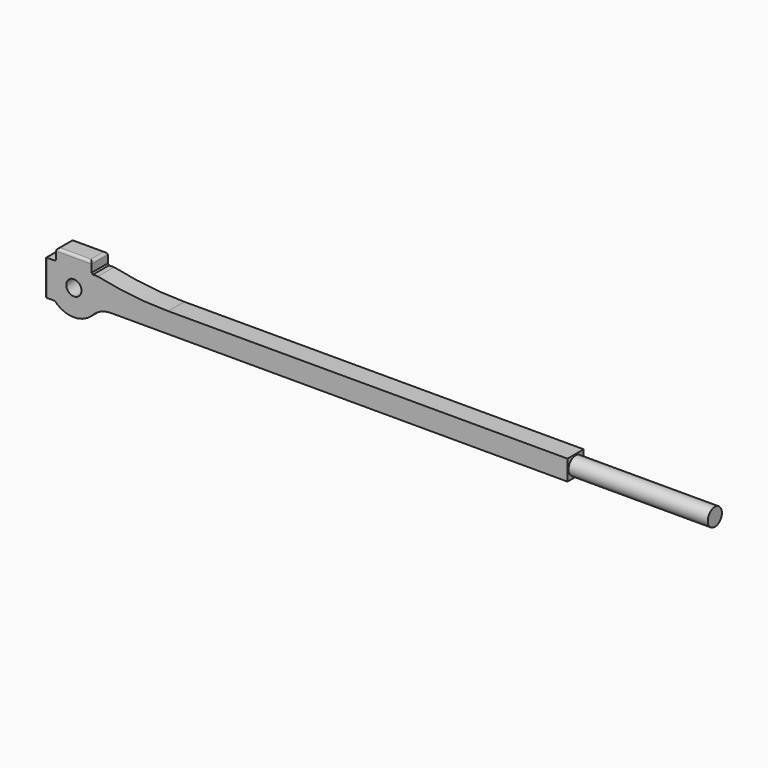
from build123d import *

# Parameters (mm, degrees)
F0_R        = 3
F1_DEPTH    = 8
F2_R        = 10
F3_T1_DEPTH = 8
F4_R        = 1
F5_R        = 3.5
F6_DEPTH    = 55


# Not quite as in the source:
# - a fillet or chamfer that OpenCascade refuses, or shapes differently, is made with other operations: its cross-section is extruded or revolved along the edge and cut away or added


with BuildPart() as f1:
    # F0 (on Front) → F1 (new body)
    with BuildSketch(Plane.XZ):
        with BuildLine():
            Line((-7.5, 7), (-11.5, 7))
            Line((-11.5, 7), (-11.5, -7))
            Line((-11.5, -7), (-7.5, -7))
            ThreePointArc((-7.5, -7), (0, -10.2591422643), (7.5, -7))
            ThreePointArc((7.5, -7), (8.6053519278, -5.5855096632), (9.4472218138, -4))
            Line((9.4472218138, -4), (9.5, -4))
            Line((9.5, -4), (195, -4))
            Line((195, -4), (195, 4))
            Line((195, 4), (9.5, 4))
            Line((9.5, 4), (9.5, 7))
            Line((9.5, 7), (7.5, 7))
            ThreePointArc((7.5, 7), (7.2543090643, 7.2543090643), (7, 7.5))
            Line((7, 7.5), (7, 11.5))
            Line((7, 11.5), (-7, 11.5))
            Line((-7, 11.5), (-7, 7.5))
            ThreePointArc((-7, 7.5), (-7.2543090643, 7.2543090643), (-7.5, 7))
        make_face()
        Circle(F0_R, mode=Mode.SUBTRACT)
    extrude(amount=F1_DEPTH)

    # F2
    f2_edges = [f1.edges().sort_by_distance(p)[0] for p in [
        (9.447222, -4, -4),
    ]]
    fillet(f2_edges, radius=F2_R)

    # F3: fillet of radius 130 on 1 edges, made by hand

    # F3_s2 → F3_t1 (join)
    with BuildSketch(Plane.XZ):
        with BuildLine():
            ThreePointArc((37.2668867538, 4), (23.3026467101, 4.7521760338), (9.5, 7))
            Line((9.5, 7), (9.5, 4))
            Line((9.5, 4), (37.2668867538, 4))
        make_face()
    extrude(amount=F3_T1_DEPTH)

    # F4
    f4_edges = [f1.edges().sort_by_distance(p)[0] for p in [
        (7, -4, 11.5),
        (-7, -4, 11.5),
        (0, 0, 11.5),
        (0, -8, 11.5),
        (-11.5, -4, 7),
        (-11.5, -4, -7),
        (-11.5, 0, 0),
        (-11.5, -8, 0),
    ]]
    fillet(f4_edges, radius=F4_R)

    # F5 (on face) → F6 (join)
    with BuildSketch(Plane.YZ.offset(195)):
        with Locations((-4, 0)):
            Circle(F5_R)
    extrude(amount=F6_DEPTH)


solid = f1.part
